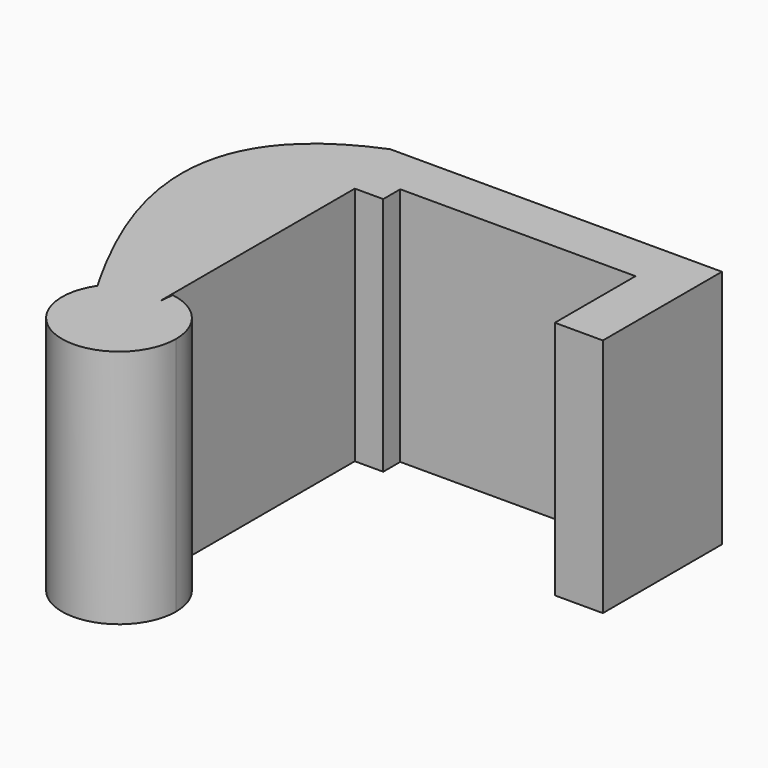
from build123d import *

# Parameters (mm, degrees)
F1_DEPTH = 25


# Not quite as in the source:
# - a feature names something its author has since deleted; it is built from what else it names


with BuildPart() as f1:
    # F0 (on Top) → F1 (new body)
    with BuildSketch(Plane.XY):
        with BuildLine():
            Line((12.25, 5.25), (12.25, -5.25))
            Line((12.25, -5.25), (17.25, -5.25))
            Line((17.25, -5.25), (17.25, 10.25))
            Line((17.25, 10.25), (-17.288029389, 10.25))
            add(Edge.make_bspline(
                [(-17.288029389, 10.25), (-33.9326616892, 3.4588538136), (-27.6432598671, -11.5939724111), (-20.8629015828, -23.4088676175)],
                knots=[0, 0, 0, 0, 33.6081495202, 33.6081495202, 33.6081495202, 33.6081495202], degree=3))
            ThreePointArc((-20.8629015828, -23.4088676175), (-18.8330680728, -21.5504075494), (-16.1829780698, -20.8080323883))
            ThreePointArc((-16.1829780698, -20.8080323883), (-15.6956355504, -20.8090410674), (-15.2100205721, -20.8500513288))
            Line((-15.2100205721, -20.8500513288), (-15.2100205721, 3.0333888489))
            Line((-15.2100205721, 3.0333888489), (-12.4874287694, 3.0333888489))
            Line((-12.4874287694, 3.0333888489), (-12.25, 5.25))
            Line((-12.25, 5.25), (12.25, 5.25))
        make_face()
        Polygon((-12.4874287694, 3.0333888489), (-12.25, 3.0333888489), (-12.25, 5.25), align=None)
        with BuildLine():
            ThreePointArc((-10.0197441457, -26.7353467643), (-10.6063091532, -24.1634313379), (-12.25, -22.1001601804))
            ThreePointArc((-12.25, -22.1001601804), (-13.5686599523, -21.3031901955), (-15.0480940947, -20.872725511))
            Line((-15.0480940947, -20.872725511), (-15.2100205721, -22.3844548448))
            Line((-15.2100205721, -22.3844548448), (-15.2100205721, -20.8500513288))
            ThreePointArc((-15.2100205721, -20.8500513288), (-15.6956355504, -20.8090410674), (-16.1829780698, -20.8080323883))
            ThreePointArc((-16.1829780698, -20.8080323883), (-18.8330680728, -21.5504075494), (-20.8629015828, -23.4088676175))
            ThreePointArc((-20.8629015828, -23.4088676175), (-17.691321516, -32.4063150838), (-10.0197441457, -26.7353467643))
        make_face()
    extrude(amount=F1_DEPTH)


solid = f1.part
